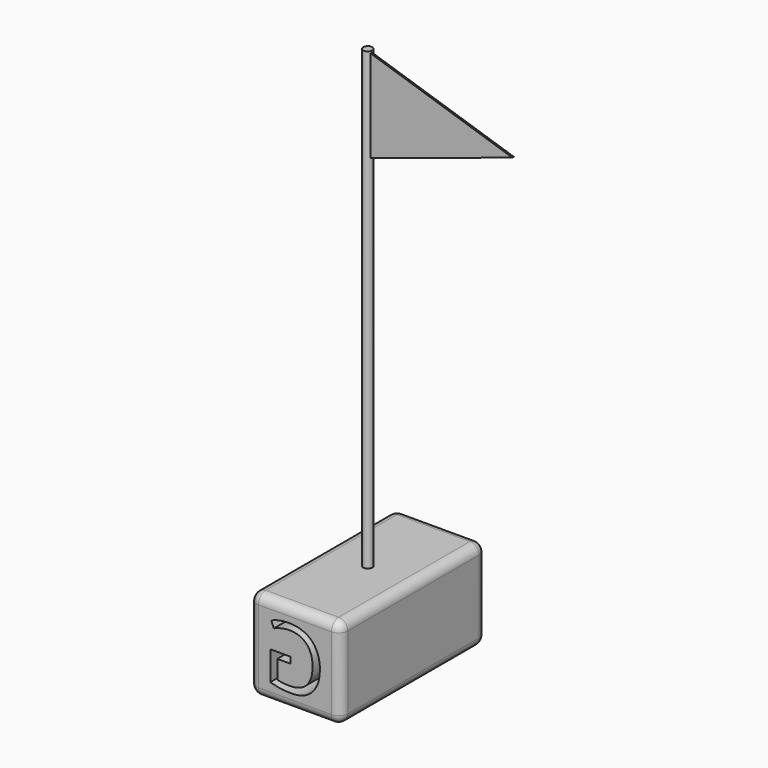
from build123d import *

# Parameters (mm, degrees)
F0_W         = 10
F0_H         = 10
F1_DEPTH     = 20
F2_R         = 1
F3_R         = 0.5
F4_DEPTH     = 50
F7_DEPTH     = 0.2
F8_TEXT_SIZE = 9.1666666667
F9_DEPTH     = 30


# Not quite as in the source:
# - Text() gives the source's letters only with a copy of the font that has no kerning and outlines rounded to 1/6400 em; it was checked with that copy


with BuildPart() as f1:
    # F0 (on Front) → F1 (new body)
    with BuildSketch(Plane.XZ):
        with Locations((5, 5)):
            Rectangle(F0_W, F0_H)
    extrude(amount=F1_DEPTH)

    # F2
    f2_edges = [f1.edges().sort_by_distance(p)[0] for p in [
        (0, -20, 5),
        (5, -20, 0),
        (10, -20, 5),
        (5, -20, 10),
        (10, -10, 0),
        (10, -10, 10),
        (10, 0, 5),
        (0, 0, 5),
        (5, 0, 0),
        (5, 0, 10),
        (0, -10, 10),
        (0, -10, 0),
    ]]
    fillet(f2_edges, radius=F2_R)

    # F3 (on face) → F4 (join)
    with BuildSketch(Plane.XY.offset(10)):
        with Locations((5, -10)):
            Circle(F3_R)
    extrude(amount=F4_DEPTH)

    # F6 (on offset) → F7 (join)
    with BuildSketch(Plane.XZ.offset(10)):
        Polygon((21.0400763899, 54.7709949315), (4.8759537749, 59.980917722), (5.0095422193, 49.510974437), align=None)
    extrude(amount=F7_DEPTH)

    # F8 (on face) → F9 (cut)
    with BuildSketch(Plane(origin=(0, 0, 0), x_dir=(-1, 0, 0), z_dir=(0, 1, 0))):
        with Locations((-8.2985677083, 1.7)):
            Text('G', F8_TEXT_SIZE, font='Open Sans', text_align=(TextAlign.LEFT, TextAlign.BOTTOM))
    extrude(amount=-F9_DEPTH, mode=Mode.SUBTRACT)


solid = f1.part
